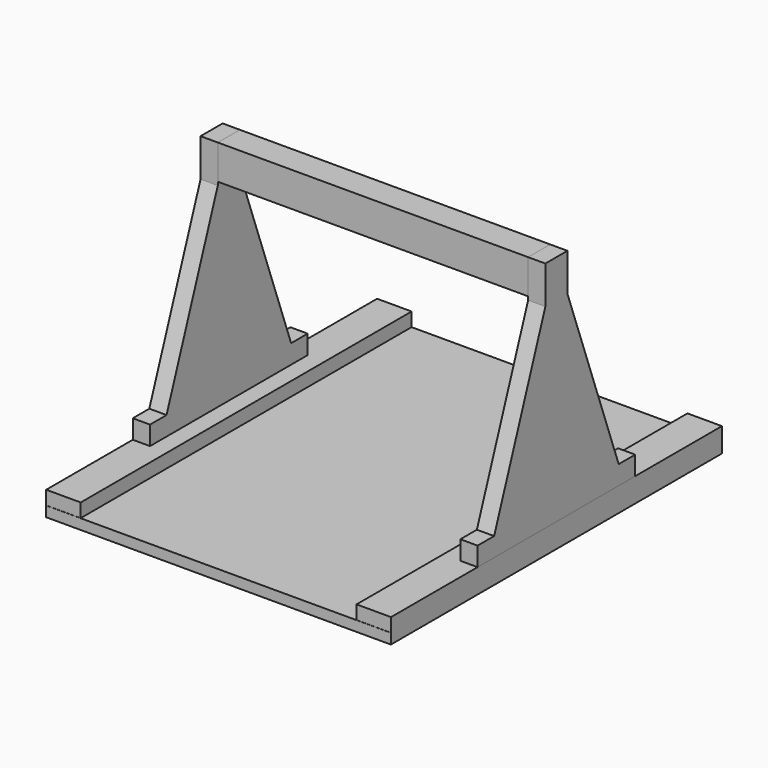
from build123d import *

# Parameters (mm, degrees)
F1_W     = 57.1539493034
F1_H     = 5
F2_DEPTH = 5
F3_DEPTH = 10
F4_DEPTH = 50
F7_DEPTH = 45


with BuildPart() as f2:
    # F1 (on offset) → F2 (new body)
    with BuildSketch(Plane.YZ.offset(-50)):
        Polygon((4, 51.0398183773), (4, 0), (22.5769746517, 0), align=None)
        Polygon((-22.5769746517, 0), (-4, 0), (-4, 51.0398183773), align=None)
        Polygon((-4, 0), (0, 0), (0, 52.0297280551), (-3.6397023427, 52.0297280551), (-4, 51.0398183773), align=None)
        Polygon((0, 52.0297280551), (0, 0), (4, 0), (4, 51.0398183773), (3.6397023427, 52.0297280551), align=None)
        Polygon((-3.6397023427, 52.0297280551), (0, 62.0297280551), (-4, 62.0297280551), (-4, 52.0297280551), align=None)
        Polygon((-3.6397023427, 52.0297280551), (0, 52.0297280551), (0, 62.0297280551), align=None)
        Polygon((4, 62.0297280551), (0, 62.0297280551), (3.6397023427, 52.0297280551), (4, 52.0297280551), align=None)
        Polygon((0, 62.0297280551), (0, 52.0297280551), (3.6397023427, 52.0297280551), align=None)
        Polygon((-4, 51.0398183773), (-3.6397023427, 52.0297280551), (-4, 52.0297280551), align=None)
        Polygon((4, 52.0297280551), (3.6397023427, 52.0297280551), (4, 51.0398183773), align=None)
        with Locations((0, -2.995375049)):
            Rectangle(F1_W, F1_H)
        Polygon((4, 0), (0, 0), (-4, 0), (-22.5769746517, 0), (-28.5769746517, 0), (-28.5769746517, -0.495375049), (28.5769746517, -0.495375049), (28.5769746517, 0), (22.5769746517, 0), align=None)
    extrude(amount=F2_DEPTH)


with BuildPart() as f3:
    # F1 (on offset) → F3 (new body)
    with BuildSketch(Plane.YZ.offset(-50)):
        Polygon((28.5769746517, -5.495375049), (-28.5769746517, -5.495375049), (-59.9543659465, -5.495375049), (-59.9543659465, -9.495375049), (60, -9.495375049), (60, -5.495375049), align=None)
    extrude(amount=F3_DEPTH)

    # F1 (on offset) → F4 (join)
    with BuildSketch(Plane.YZ.offset(-50)):
        Polygon((60, -9.495375049), (-59.9543659465, -9.495375049), (-60, -9.495375049), (-60, -12.4950279511), (60, -12.4950279511), align=None)
    extrude(amount=F4_DEPTH)

    # F9: F3 across plane


with BuildPart() as f7:
    # F6 (on offset) → F7 (new body)
    with BuildSketch(Plane.YZ.offset(-45)):
        Polygon((3.5, 52.5297280551), (4, 52.0297280551), (4, 57.0297280551), (3.5, 57.0297280551), align=None)
        Polygon((0, 52.0297280551), (4, 52.0297280551), (3.5, 52.5297280551), (0, 52.5297280551), align=None)
        Polygon((-4, 52.0297280551), (0, 52.0297280551), (0, 52.5297280551), (-3.5, 52.5297280551), align=None)
        Polygon((3.5, 57.0297280551), (4, 57.0297280551), (4, 62.0297280551), (3.5, 61.5297280551), align=None)
        Polygon((-4, 57.0297280551), (-4, 52.0297280551), (-3.5, 52.5297280551), (-3.5, 57.0297280551), align=None)
        Polygon((3.5, 61.5297280551), (4, 62.0297280551), (0, 62.0297280551), (0, 61.5297280551), align=None)
        Polygon((-4, 62.0297280551), (-4, 57.0297280551), (-3.5, 57.0297280551), (-3.5, 61.5297280551), align=None)
        Polygon((0, 61.5297280551), (0, 62.0297280551), (-4, 62.0297280551), (-3.5, 61.5297280551), align=None)
    extrude(amount=F7_DEPTH)

    # F10: F7 across plane


with BuildPart() as f8_1:
    # F8: instance of F2
    add(f2.part.mirror(Plane.YZ))


with BuildPart() as f3_1:
    add(f3.part)
    add(f3.part.mirror(Plane.YZ))


with BuildPart() as f7_1:
    add(f7.part)
    add(f7.part.mirror(Plane.YZ))


solid = Compound([f2.part, f8_1.part, f3_1.part, f7_1.part])
